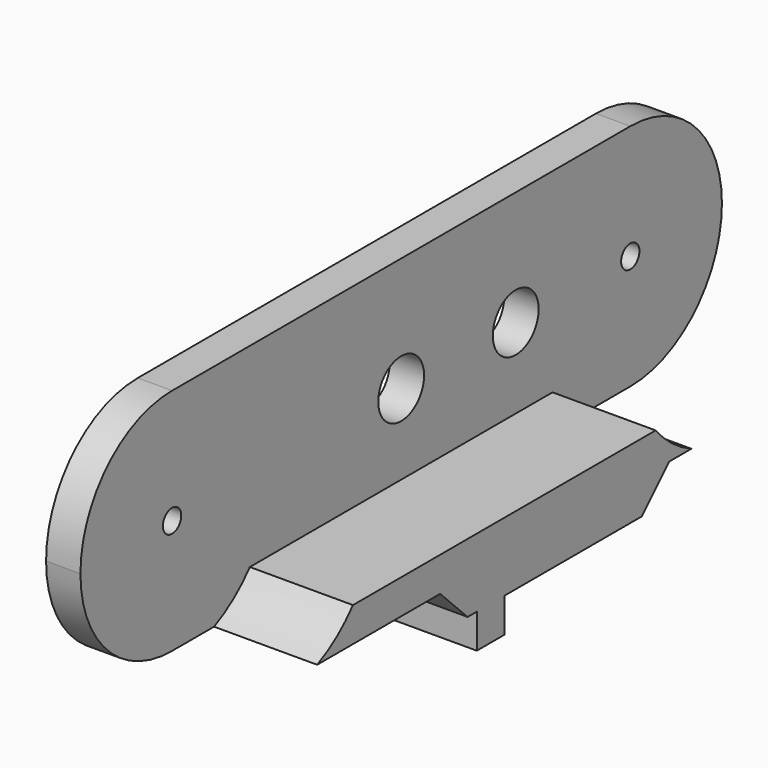
from build123d import *

# Parameters (mm, degrees)
F0_W      = 70
F0_H      = 20
F1_DEPTH  = 3
F3_DEPTH  = 9
F5_DEPTH  = 25
F6_R      = 1
F7_DEPTH  = 25
F8_R      = 2.5
F9_DEPTH  = 25
F10_W     = 3
F10_H     = 3
F11_DEPTH = 12
F12_SIZE  = 2.99999


# Not quite as in the source:
# - a fillet or chamfer is up to 0.001 mm smaller than in the source, because OpenCascade refuses the exact size


with BuildPart() as f1:
    # F0 (on Right) → F1 (new body)
    with BuildSketch(Plane.YZ):
        with Locations((15.2043993567, 29.5881517231)):
            Rectangle(F0_W, F0_H)
    extrude(amount=F1_DEPTH)

    # F2 (on face) → F3 (join)
    with BuildSketch(Plane.YZ.offset(3)):
        with BuildLine():
            ThreePointArc((-1.3103192691, 22.5881517231), (-3.0917046048, 20.8670406755), (-5.2130249484, 19.5881517231))
            Line((-5.2130249484, 19.5881517231), (0.2043993567, 19.5881517231))
            Line((0.2043993567, 19.5881517231), (0.2043993567, 22.5881517231))
            Line((0.2043993567, 22.5881517231), (-1.3103192691, 22.5881517231))
        make_face()
        with BuildLine():
            Line((0.2043993567, 22.5881517231), (0.2043993567, 19.5881517231))
            Line((0.2043993567, 19.5881517231), (35.6218236617, 19.5881517231))
            ThreePointArc((35.6218236617, 19.5881517231), (33.5005033181, 20.8670406755), (31.7191179824, 22.5881517231))
            Line((31.7191179824, 22.5881517231), (0.2043993567, 22.5881517231))
        make_face()
    extrude(amount=F3_DEPTH)

    # F4 (on face) → F5 (cut)
    with BuildSketch(Plane(origin=(0, 0, 0), x_dir=(0, -1, 0), z_dir=(-1, 0, 0))):
        with BuildLine():
            Line((19.7956006433, 29.5881517231), (19.7956006433, 39.5881517231))
            Line((19.7956006433, 39.5881517231), (9.7956006433, 39.5881517231))
            ThreePointArc((9.7956006433, 39.5881517231), (16.8666684552, 36.659219535), (19.7956006433, 29.5881517231))
        make_face()
        with BuildLine():
            Line((19.7956006433, 19.5881517231), (19.7956006433, 29.5881517231))
            ThreePointArc((19.7956006433, 29.5881517231), (16.8666684552, 22.5170839113), (9.7956006433, 19.5881517231))
            Line((9.7956006433, 19.5881517231), (19.7956006433, 19.5881517231))
        make_face()
        with BuildLine():
            ThreePointArc((-50.2043993567, 29.5881517231), (-47.2754671685, 36.659219535), (-40.2043993567, 39.5881517231))
            Line((-40.2043993567, 39.5881517231), (-50.2043993567, 39.5881517231))
            Line((-50.2043993567, 39.5881517231), (-50.2043993567, 29.5881517231))
        make_face()
        with BuildLine():
            ThreePointArc((-40.2043993567, 19.5881517231), (-47.2754671685, 22.5170839113), (-50.2043993567, 29.5881517231))
            Line((-50.2043993567, 29.5881517231), (-50.2043993567, 19.5881517231))
            Line((-50.2043993567, 19.5881517231), (-40.2043993567, 19.5881517231))
        make_face()
    extrude(amount=-F5_DEPTH, mode=Mode.SUBTRACT)

    # F6 (on face) → F7 (cut)
    with BuildSketch(Plane.YZ.offset(3)):
        with Locations((-9.7956006433, 29.5881517231)):
            Circle(F6_R)
        with Locations((40.2043993567, 29.5881517231)):
            Circle(F6_R)
    extrude(amount=-F7_DEPTH, mode=Mode.SUBTRACT)

    # F8 (on face) → F9 (cut)
    with BuildSketch(Plane(origin=(0, 0, 0), x_dir=(0, -1, 0), z_dir=(-1, 0, 0))):
        with Locations((-27.7043993567, 29.5881517231)):
            Circle(F8_R)
        with Locations((-15.2043993567, 29.5881517231)):
            Circle(F8_R)
    extrude(amount=-F9_DEPTH, mode=Mode.SUBTRACT)

    # F10 (on face) → F11 (join)
    with BuildSketch(Plane(origin=(0, 0, 0), x_dir=(0, -1, 0), z_dir=(-1, 0, 0))):
        Polygon((-8.2043993567, 16.5881517231), (-8.2043993567, 19.5881517231), (-33.2043993567, 19.5881517231), (-33.2043993567, 16.5881517231), (-15.2043993567, 16.5881517231), (-12.2043993567, 16.5881517231), align=None)
        with Locations((-13.7043993567, 15.0881517231)):
            Rectangle(F10_W, F10_H)
    extrude(amount=-F11_DEPTH)

    # F12 (size 3 in the source; OpenCascade refuses exactly that, so slightly less here)
    f12_edges = [f1.edges().sort_by_distance(p)[0] for p in [
        (6, 8.204399, 16.588152),
        (6, 33.204399, 16.588152),
    ]]
    chamfer(f12_edges, length=F12_SIZE)


solid = f1.part
